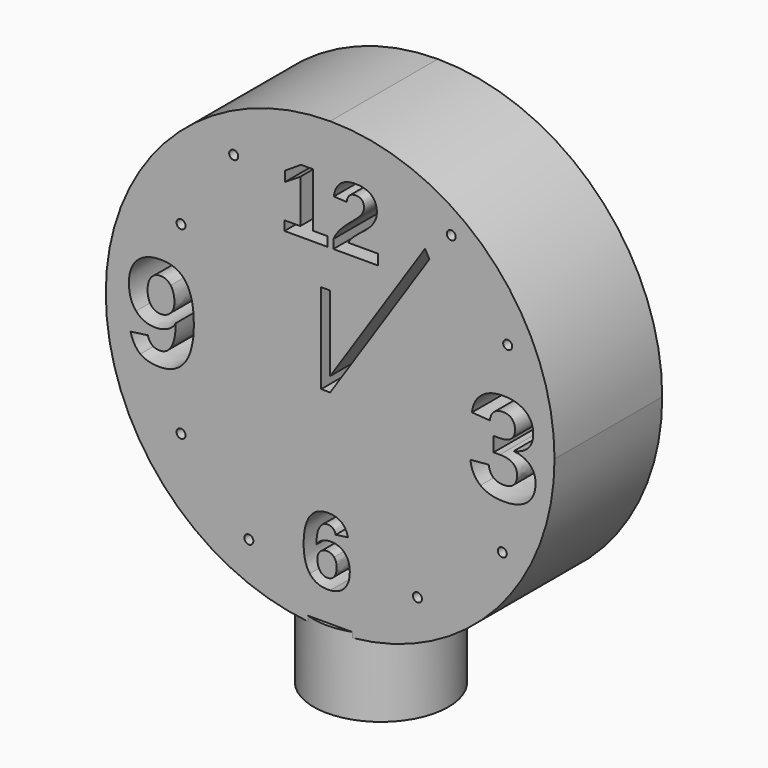
from build123d import *

# Parameters (mm, degrees)
F1_DEPTH = 15
F0_R     = 0.5
F3_START = -24.3
F2_R     = 7.5
F3_DEPTH = 8.6


with BuildPart() as f1:
    # F0 (on Front) → F1 (new body)
    with BuildSketch(Plane.XZ):
        with BuildLine():
            add(Edge.make_bspline(
                [(-17.7850674081, 0.4010269896), (-17.3510803997, 0.8501802107), (-17.3510803997, 1.6014910531)],
                knots=[0, 0, 0, 1, 1, 1], degree=2))
            add(Edge.make_bspline(
                [(-17.3510803997, 1.6014910531), (-17.3510803997, 2.5557958188), (-17.7710678272, 3.1204455824)],
                knots=[0, 0, 0, 1, 1, 1], degree=2))
            add(Edge.make_bspline(
                [(-17.7710678272, 3.1204455824), (-18.1910552546, 3.6850953459), (-18.8817012465, 3.6850953459)],
                knots=[0, 0, 0, 1, 1, 1], degree=2))
            add(Edge.make_bspline(
                [(-18.8817012465, 3.6850953459), (-19.5606809208, 3.6850953459), (-19.950335923, 3.1927767504)],
                knots=[0, 0, 0, 1, 1, 1], degree=2))
            add(Edge.make_bspline(
                [(-19.950335923, 3.1927767504), (-20.3399909251, 2.7004581549), (-20.3399909251, 1.8348174017)],
                knots=[0, 0, 0, 1, 1, 1], degree=2))
            add(Edge.make_bspline(
                [(-20.3399909251, 1.8348174017), (-20.3399909251, 0.9808429659), (-19.9538358182, 0.4663583672)],
                knots=[0, 0, 0, 1, 1, 1], degree=2))
            add(Edge.make_bspline(
                [(-19.9538358182, 0.4663583672), (-19.5676807113, -0.0481262314), (-18.874701456, -0.0481262314)],
                knots=[0, 0, 0, 1, 1, 1], degree=2))
            add(Edge.make_bspline(
                [(-18.874701456, -0.0481262314), (-18.2190544165, -0.0481262314), (-17.7850674081, 0.4010269896)],
                knots=[0, 0, 0, 1, 1, 1], degree=2))
        make_face()
    extrude(amount=F1_DEPTH)


with BuildPart() as f1b:
    # F0 (on Front) → F1, piece 2 (new body)
    with BuildSketch(Plane.XZ):
        with BuildLine():
            add(Edge.make_bspline(
                [(0.4478049096, -19.5360259002), (0.722932181, -19.1852594091), (0.722932181, -18.5668464486)],
                knots=[0, 0, 0, 1, 1, 1], degree=2))
            add(Edge.make_bspline(
                [(0.722932181, -18.5668464486), (0.722932181, -17.9434462868), (0.4345057061, -17.6134598012)],
                knots=[0, 0, 0, 1, 1, 1], degree=2))
            add(Edge.make_bspline(
                [(0.4345057061, -17.6134598012), (0.1460792312, -17.2834733155), (-0.3576280995, -17.2834733155)],
                knots=[0, 0, 0, 1, 1, 1], degree=2))
            add(Edge.make_bspline(
                [(-0.3576280995, -17.2834733155), (-0.8413866251, -17.2834733155), (-1.1323067006, -17.5926797958)],
                knots=[0, 0, 0, 1, 1, 1], degree=2))
            add(Edge.make_bspline(
                [(-1.1323067006, -17.5926797958), (-1.4232267761, -17.901886276), (-1.4232267761, -18.4122432085)],
                knots=[0, 0, 0, 1, 1, 1], degree=2))
            add(Edge.make_bspline(
                [(-1.4232267761, -18.4122432085), (-1.4232267761, -19.0506049742), (-1.1190074971, -19.4686986827)],
                knots=[0, 0, 0, 1, 1, 1], degree=2))
            add(Edge.make_bspline(
                [(-1.1190074971, -19.4686986827), (-0.8147882182, -19.8867923912), (-0.32105529, -19.8867923912)],
                knots=[0, 0, 0, 1, 1, 1], degree=2))
            add(Edge.make_bspline(
                [(-0.32105529, -19.8867923912), (0.1726776382, -19.8867923912), (0.4478049096, -19.5360259002)],
                knots=[0, 0, 0, 1, 1, 1], degree=2))
        make_face()
    extrude(amount=F1_DEPTH)


with BuildPart() as f1c:
    # F0 (on Front) → F1, piece 3 (new body)
    with BuildSketch(Plane.XZ):
        with BuildLine():
            ThreePointArc((0, -25), (17.6776695297, -17.6776695297), (25, 0))
            ThreePointArc((25, 0), (17.6776695297, 17.6776695297), (0, 25))
            ThreePointArc((0, 25), (-17.6776695297, 17.6776695297), (-25, 0))
            ThreePointArc((-25, 0), (-17.6776695297, -17.6776695297), (0, -25))
        make_face()
        with Locations((-9.0576551073, -18.9760137498)):
            Circle(F0_R, mode=Mode.SUBTRACT)
        with BuildLine():
            add(Edge.make_bspline(
                [(1.5333523913, -20.359745314), (0.9591361314, -20.9441763485), (0, -21.0155943762)],
                knots=[0, 0, 0, 0.8777990499, 0.8777990499, 0.8777990499], degree=2))
            add(Edge.make_bspline(
                [(0, -21.0155943762), (-0.1335241209, -21.0255366868), (-0.2745080779, -21.0255366868)],
                knots=[0.8777990499, 0.8777990499, 0.8777990499, 1, 1, 1], degree=2))
            add(Edge.make_bspline(
                [(-0.2745080779, -21.0255366868), (-1.5678556136, -21.0255366868), (-2.2619077938, -20.1186972514)],
                knots=[0, 0, 0, 1, 1, 1], degree=2))
            add(Edge.make_bspline(
                [(-2.2619077938, -20.1186972514), (-2.9559599739, -19.211857816), (-2.9559599739, -17.4297645535)],
                knots=[0, 0, 0, 1, 1, 1], degree=2))
            add(Edge.make_bspline(
                [(-2.9559599739, -17.4297645535), (-2.9559599739, -15.4714568452), (-2.2519333912, -14.4814973882)],
                knots=[0, 0, 0, 1, 1, 1], degree=2))
            add(Edge.make_bspline(
                [(-2.2519333912, -14.4814973882), (-1.5479068084, -13.4915379313), (-0.2379352684, -13.4915379313)],
                knots=[0, 0, 0, 1, 1, 1], degree=2))
            add(Edge.make_bspline(
                [(-0.2379352684, -13.4915379313), (0.6913465728, -13.4915379313), (1.2291331124, -13.9021508379)],
                knots=[0, 0, 0, 1, 1, 1], degree=2))
            add(Edge.make_bspline(
                [(1.2291331124, -13.9021508379), (1.766919652, -14.3127637444), (1.9896813098, -15.1755495684)],
                knots=[0, 0, 0, 1, 1, 1], degree=2))
            Line((1.9896813098, -15.1755495684), (0.6132137525, -15.366725618))
            add(Edge.make_bspline(
                [(0.6132137525, -15.366725618), (0.4170505016, -14.6452438307), (-0.2695208766, -14.6452438307)],
                knots=[0, 0, 0, 1, 1, 1], degree=2))
            add(Edge.make_bspline(
                [(-0.2695208766, -14.6452438307), (-0.8563482289, -14.6452438307), (-1.1913219159, -15.232071183)],
                knots=[0, 0, 0, 1, 1, 1], degree=2))
            add(Edge.make_bspline(
                [(-1.1913219159, -15.232071183), (-1.5262956028, -15.8188985354), (-1.5262956028, -17.0141644456)],
                knots=[0, 0, 0, 1, 1, 1], degree=2))
            add(Edge.make_bspline(
                [(-1.5262956028, -17.0141644456), (-1.2935595424, -16.6251627446), (-0.8779594346, -16.4173626907)],
                knots=[0, 0, 0, 1, 1, 1], degree=2))
            add(Edge.make_bspline(
                [(-0.8779594346, -16.4173626907), (-0.4623593267, -16.2095626368), (0.0629592097, -16.2095626368)],
                knots=[0, 0, 0, 1, 1, 1], degree=2))
            add(Edge.make_bspline(
                [(0.0629592097, -16.2095626368), (1.0454378647, -16.2095626368), (1.6164724129, -16.8329627986)],
                knots=[0, 0, 0, 1, 1, 1], degree=2))
            add(Edge.make_bspline(
                [(1.6164724129, -16.8329627986), (2.1875069611, -17.4563629604), (2.1875069611, -18.5252864378)],
                knots=[0, 0, 0, 1, 1, 1], degree=2))
            add(Edge.make_bspline(
                [(2.1875069611, -18.5252864378), (2.1875069611, -19.6939539412), (1.5333523913, -20.359745314)],
                knots=[0, 0, 0, 1, 1, 1], degree=2))
        make_face(mode=Mode.SUBTRACT)
        with Locations((-16.6161694347, -11.0553130187)):
            Circle(F0_R, mode=Mode.SUBTRACT)
        with Locations((9.7307167873, -18.537102893)):
            Circle(F0_R, mode=Mode.SUBTRACT)
        with Locations((19.1797496622, -11.0553130187)):
            Circle(F0_R, mode=Mode.SUBTRACT)
        with BuildLine():
            add(Edge.make_bspline(
                [(22.2598520542, -1.472298656), (22.8838185625, -2.0962651643), (22.8838185625, -3.0658657712)],
                knots=[0, 0, 0, 1, 1, 1], degree=2))
            add(Edge.make_bspline(
                [(22.8838185625, -3.0658657712), (22.8838185625, -4.4780605376), (21.9575648061, -5.2480374902)],
                knots=[0, 0, 0, 1, 1, 1], degree=2))
            add(Edge.make_bspline(
                [(21.9575648061, -5.2480374902), (21.0313110498, -6.0180144428), (19.3202511552, -6.0180144428)],
                knots=[0, 0, 0, 1, 1, 1], degree=2))
            add(Edge.make_bspline(
                [(19.3202511552, -6.0180144428), (17.7004477882, -6.0180144428), (16.745676367, -5.2731330353)],
                knots=[0, 0, 0, 1, 1, 1], degree=2))
            add(Edge.make_bspline(
                [(16.745676367, -5.2731330353), (15.7909049458, -4.5282516279), (15.6266431959, -3.1229011011)],
                knots=[0, 0, 0, 1, 1, 1], degree=2))
            Line((15.6266431959, -3.1229011011), (17.6662265903, -2.944950872))
            add(Edge.make_bspline(
                [(17.6662265903, -2.944950872), (17.8578652985, -4.3913668363), (19.3134069156, -4.3913668363)],
                knots=[0, 0, 0, 1, 1, 1], degree=2))
            add(Edge.make_bspline(
                [(19.3134069156, -4.3913668363), (20.0320520714, -4.3913668363), (20.4312993801, -4.0354663782)],
                knots=[0, 0, 0, 1, 1, 1], degree=2))
            add(Edge.make_bspline(
                [(20.4312993801, -4.0354663782), (20.8305466889, -3.6795659201), (20.8305466889, -2.944950872)],
                knots=[0, 0, 0, 1, 1, 1], degree=2))
            add(Edge.make_bspline(
                [(20.8305466889, -2.944950872), (20.8305466889, -2.2742153933), (20.3457463854, -1.9183149352)],
                knots=[0, 0, 0, 1, 1, 1], degree=2))
            add(Edge.make_bspline(
                [(20.3457463854, -1.9183149352), (19.8609460819, -1.5624144771), (18.9050339541, -1.5624144771)],
                knots=[0, 0, 0, 1, 1, 1], degree=2))
            Line((18.9050339541, -1.5624144771), (18.206921517, -1.5624144771))
            Line((18.206921517, -1.5624144771), (18.206921517, 0.0573888898))
            Line((18.206921517, 0.0573888898), (18.8639685166, 0.0573888898))
            add(Edge.make_bspline(
                [(18.8639685166, 0.0573888898), (19.7263427035, 0.0573888898), (20.1609519168, 0.4098672281)],
                knots=[0, 0, 0, 1, 1, 1], degree=2))
            add(Edge.make_bspline(
                [(20.1609519168, 0.4098672281), (20.59556113, 0.7623455664), (20.59556113, 1.419392566)],
                knots=[0, 0, 0, 1, 1, 1], degree=2))
            add(Edge.make_bspline(
                [(20.59556113, 1.419392566), (20.59556113, 2.0376555412), (20.2499270313, 2.3912745861)],
                knots=[0, 0, 0, 1, 1, 1], degree=2))
            add(Edge.make_bspline(
                [(20.2499270313, 2.3912745861), (19.9042929326, 2.744893631), (19.2404016934, 2.744893631)],
                knots=[0, 0, 0, 1, 1, 1], degree=2))
            add(Edge.make_bspline(
                [(19.2404016934, 2.744893631), (18.619857305, 2.744893631), (18.2388613017, 2.4026816521)],
                knots=[0, 0, 0, 1, 1, 1], degree=2))
            add(Edge.make_bspline(
                [(18.2388613017, 2.4026816521), (17.8578652985, 2.0604696732), (17.8008299687, 1.4330810451)],
                knots=[0, 0, 0, 1, 1, 1], degree=2))
            Line((17.8008299687, 1.4330810451), (15.7977491854, 1.5745286631))
            add(Edge.make_bspline(
                [(15.7977491854, 1.5745286631), (15.9551666957, 2.8726527698), (16.8745762124, 3.6072678179)],
                knots=[0, 0, 0, 1, 1, 1], degree=2))
            add(Edge.make_bspline(
                [(16.8745762124, 3.6072678179), (17.7939857291, 4.3418828661), (19.2769043045, 4.3418828661)],
                knots=[0, 0, 0, 1, 1, 1], degree=2))
            add(Edge.make_bspline(
                [(19.2769043045, 4.3418828661), (20.8533608208, 4.3418828661), (21.7408305528, 3.6323633631)],
                knots=[0, 0, 0, 1, 1, 1], degree=2))
            add(Edge.make_bspline(
                [(21.7408305528, 3.6323633631), (22.6283002849, 2.9228438601), (22.6283002849, 1.668066604)],
                knots=[0, 0, 0, 1, 1, 1], degree=2))
            add(Edge.make_bspline(
                [(22.6283002849, 1.668066604), (22.6283002849, 0.7258429553), (22.0750575856, 0.1201277526)],
                knots=[0, 0, 0, 1, 1, 1], degree=2))
            add(Edge.make_bspline(
                [(22.0750575856, 0.1201277526), (21.5218148863, -0.4855874501), (20.4814904704, -0.6840703979)],
                knots=[0, 0, 0, 1, 1, 1], degree=2))
            Line((20.4814904704, -0.6840703979), (20.4814904704, -0.7137287694))
            add(Edge.make_bspline(
                [(20.4814904704, -0.7137287694), (21.6358855459, -0.8483321477), (22.2598520542, -1.472298656)],
                knots=[0, 0, 0, 1, 1, 1], degree=2))
        make_face(mode=Mode.SUBTRACT)
        with BuildLine():
            add(Edge.make_bspline(
                [(-16.0864515904, 4.0105856022), (-15.1858118849, 2.7307905802), (-15.1858118849, 0.1642007458)],
                knots=[0, 0, 0, 1, 1, 1], degree=2))
            add(Edge.make_bspline(
                [(-15.1858118849, 0.1642007458), (-15.1858118849, -2.5703840596), (-16.1844486568, -3.9271767766)],
                knots=[0, 0, 0, 1, 1, 1], degree=2))
            add(Edge.make_bspline(
                [(-16.1844486568, -3.9271767766), (-17.1830854288, -5.2839694936), (-19.0216970556, -5.2839694936)],
                knots=[0, 0, 0, 1, 1, 1], degree=2))
            add(Edge.make_bspline(
                [(-19.0216970556, -5.2839694936), (-20.3773231409, -5.2839694936), (-21.1461334594, -4.7041535173)],
                knots=[0, 0, 0, 1, 1, 1], degree=2))
            add(Edge.make_bspline(
                [(-21.1461334594, -4.7041535173), (-21.914943778, -4.1243375411), (-22.2369341391, -2.8690417857)],
                knots=[0, 0, 0, 1, 1, 1], degree=2))
            Line((-22.2369341391, -2.8690417857), (-20.3119917633, -2.5983832214))
            add(Edge.make_bspline(
                [(-20.3119917633, -2.5983832214), (-20.027333618, -3.6716844249), (-18.9983644207, -3.6716844249)],
                knots=[0, 0, 0, 1, 1, 1], degree=2))
            add(Edge.make_bspline(
                [(-18.9983644207, -3.6716844249), (-18.139723458, -3.6716844249), (-17.676570656, -2.8480424144)],
                knots=[0, 0, 0, 1, 1, 1], degree=2))
            add(Edge.make_bspline(
                [(-17.676570656, -2.8480424144), (-17.2134178541, -2.0244004039), (-17.1994182732, -0.4051155447)],
                knots=[0, 0, 0, 1, 1, 1], degree=2))
            add(Edge.make_bspline(
                [(-17.1994182732, -0.4051155447), (-17.4747433645, -0.9510992004), (-18.1058911374, -1.261423244)],
                knots=[0, 0, 0, 1, 1, 1], degree=2))
            add(Edge.make_bspline(
                [(-18.1058911374, -1.261423244), (-18.7370389103, -1.5717472876), (-19.4650171179, -1.5717472876)],
                knots=[0, 0, 0, 1, 1, 1], degree=2))
            add(Edge.make_bspline(
                [(-19.4650171179, -1.5717472876), (-20.8229764667, -1.5717472876), (-21.6209525788, -0.648941579)],
                knots=[0, 0, 0, 1, 1, 1], degree=2))
            add(Edge.make_bspline(
                [(-21.6209525788, -0.648941579), (-22.418928691, 0.2738641297), (-22.418928691, 1.8488169826)],
                knots=[0, 0, 0, 1, 1, 1], degree=2))
            add(Edge.make_bspline(
                [(-22.418928691, 1.8488169826), (-22.418928691, 3.4681018418), (-21.4821234014, 4.379241233)],
                knots=[0, 0, 0, 1, 1, 1], degree=2))
            add(Edge.make_bspline(
                [(-21.4821234014, 4.379241233), (-20.5453181118, 5.2903806242), (-18.8327027132, 5.2903806242)],
                knots=[0, 0, 0, 1, 1, 1], degree=2))
            add(Edge.make_bspline(
                [(-18.8327027132, 5.2903806242), (-16.987091296, 5.2903806242), (-16.0864515904, 4.0105856022)],
                knots=[0, 0, 0, 1, 1, 1], degree=2))
        make_face(mode=Mode.SUBTRACT)
        with Locations((-16.6161694347, 9.4938481434)):
            Circle(F0_R, mode=Mode.SUBTRACT)
        with Locations((-10.7461412923, 18.1974526392)):
            Circle(F0_R, mode=Mode.SUBTRACT)
        Polygon((-0.288864803, 12.5784629583), (-5.0851619623, 12.5784629583), (-5.0851619623, 13.6301694879), (-3.3280228754, 13.6301694879), (-3.3280228754, 18.4667310626), (-5.0287917807, 17.4053610733), (-5.0287917807, 18.5182695143), (-3.2523257745, 19.6698317939), (-1.9139366074, 19.6698317939), (-1.9139366074, 13.6301694879), (-0.288864803, 13.6301694879), align=None, mode=Mode.SUBTRACT)
        Polygon((0, 8.3937322441), (0, 0), (10.571134303, 15.9335022082), (11.0569010444, 15.0594137271), (0, -1.6062677559), (-1, -1.6062677559), (-1, 8.3937322441), align=None, mode=Mode.SUBTRACT)
        with Locations((19.7811665086, 9.4938481434)):
            Circle(F0_R, mode=Mode.SUBTRACT)
        with BuildLine():
            Line((5.3175523937, 12.5784629583), (0.355365843, 12.5784629583))
            Line((0.355365843, 12.5784629583), (0.355365843, 13.5593041168))
            add(Edge.make_bspline(
                [(0.355365843, 13.5593041168), (0.6323850208, 14.1697126539), (1.1429378077, 14.7479096587)],
                knots=[0, 0, 0, 1, 1, 1], degree=2))
            add(Edge.make_bspline(
                [(1.1429378077, 14.7479096587), (1.6534905947, 15.3261066634), (2.4281779465, 15.9558421199)],
                knots=[0, 0, 0, 1, 1, 1], degree=2))
            add(Edge.make_bspline(
                [(2.4281779465, 15.9558421199), (3.1738749192, 16.5598083505), (3.4734421696, 16.9519837562)],
                knots=[0, 0, 0, 1, 1, 1], degree=2))
            add(Edge.make_bspline(
                [(3.4734421696, 16.9519837562), (3.7730094199, 17.344159162), (3.7730094199, 17.7226446665)],
                knots=[0, 0, 0, 1, 1, 1], degree=2))
            add(Edge.make_bspline(
                [(3.7730094199, 17.7226446665), (3.7730094199, 18.6487262201), (2.8420961365, 18.6487262201)],
                knots=[0, 0, 0, 1, 1, 1], degree=2))
            add(Edge.make_bspline(
                [(2.8420961365, 18.6487262201), (2.3879135311, 18.6487262201), (2.1495481921, 18.4047238629)],
                knots=[0, 0, 0, 1, 1, 1], degree=2))
            add(Edge.make_bspline(
                [(2.1495481921, 18.4047238629), (1.9111828531, 18.1607215057), (1.840317482, 17.6727167914)],
                knots=[0, 0, 0, 1, 1, 1], degree=2))
            Line((1.840317482, 17.6727167914), (0.4149571778, 17.7532456222))
            add(Edge.make_bspline(
                [(0.4149571778, 17.7532456222), (0.5357504239, 18.7389185105), (1.1526012674, 19.2575241805)],
                knots=[0, 0, 0, 1, 1, 1], degree=2))
            add(Edge.make_bspline(
                [(1.1526012674, 19.2575241805), (1.7694521109, 19.7761298505), (2.8308221002, 19.7761298505)],
                knots=[0, 0, 0, 1, 1, 1], degree=2))
            add(Edge.make_bspline(
                [(2.8308221002, 19.7761298505), (3.9791632266, 19.7761298505), (4.5927929169, 19.2526924507)],
                knots=[0, 0, 0, 1, 1, 1], degree=2))
            add(Edge.make_bspline(
                [(4.5927929169, 19.2526924507), (5.2064226072, 18.7292550508), (5.2064226072, 17.7822360012)],
                knots=[0, 0, 0, 1, 1, 1], degree=2))
            add(Edge.make_bspline(
                [(5.2064226072, 17.7822360012), (5.2064226072, 17.2845678272), (5.0107375485, 16.8819236735)],
                knots=[0, 0, 0, 1, 1, 1], degree=2))
            add(Edge.make_bspline(
                [(5.0107375485, 16.8819236735), (4.8150524898, 16.4792795197), (4.5074323563, 16.139447854)],
                knots=[0, 0, 0, 1, 1, 1], degree=2))
            add(Edge.make_bspline(
                [(4.5074323563, 16.139447854), (4.1998122229, 15.7996161882), (3.8253531599, 15.5024648028)],
                knots=[0, 0, 0, 1, 1, 1], degree=2))
            add(Edge.make_bspline(
                [(3.8253531599, 15.5024648028), (3.4508940969, 15.2053134173), (3.0981778183, 14.9234625097)],
                knots=[0, 0, 0, 1, 1, 1], degree=2))
            add(Edge.make_bspline(
                [(3.0981778183, 14.9234625097), (2.7454615396, 14.6416116021), (2.4563630372, 14.3549289646)],
                knots=[0, 0, 0, 1, 1, 1], degree=2))
            add(Edge.make_bspline(
                [(2.4563630372, 14.3549289646), (2.1672645348, 14.0682463272), (2.0255337927, 13.7412992743)],
                knots=[0, 0, 0, 1, 1, 1], degree=2))
            Line((2.0255337927, 13.7412992743), (5.3175523937, 13.7412992743))
            Line((5.3175523937, 13.7412992743), (5.3175523937, 12.5784629583))
        make_face(mode=Mode.SUBTRACT)
        with Locations((13.4934755042, 18.1974526392)):
            Circle(F0_R, mode=Mode.SUBTRACT)
    extrude(amount=F1_DEPTH)

    # F2 (on Top) → F3 (join)
    with BuildSketch(Plane.XY.offset(F3_START)):
        with Locations((0, -7.9162725751)):
            Circle(F2_R)
    extrude(amount=-F3_DEPTH)


solid = Compound([f1.part, f1b.part, f1c.part])
